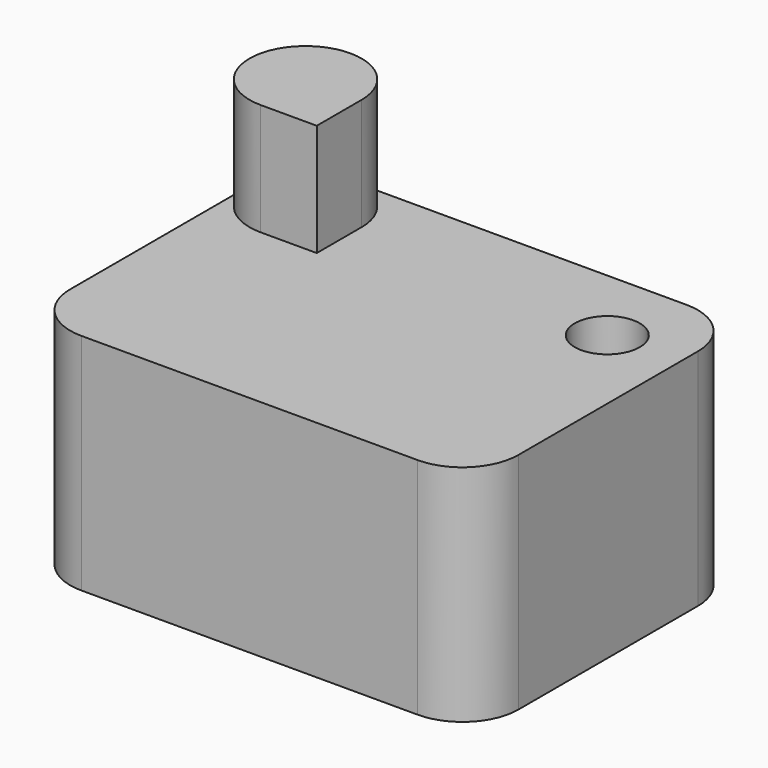
from build123d import *
from build123d import SkipClean  # not in build123d's __all__

# Parameters (mm, degrees)
F0_W      = 101.6
F0_H      = 76.2
F1_DEPTH  = 50.8
F2_R      = 12.7
F4_DEPTH  = 25.4
F9_R      = 7.3504137181
F10_DEPTH = 25.4


# Not quite as in the source:
# - after a boolean that leaves OpenCascade's solid faulty, fix() repairs it
# - the program builds the solid bodies; features that only make, move or delete a surface that nothing else refers to are left out


with BuildPart() as f1:
    # F0 (on Top) → F1 (new body)
    with BuildSketch(Plane.XY):
        with Locations((50.8, 38.1)):
            Rectangle(F0_W, F0_H)
    extrude(amount=F1_DEPTH)

    # F2
    f2_edges = [f1.edges().sort_by_distance(p)[0] for p in [
        (0, 0, 25.4),
        (101.6, 0, 25.4),
        (101.6, 76.2, 25.4),
        (0, 76.2, 25.4),
    ]]
    fillet(f2_edges, radius=F2_R)

    # F3 (on face) → F4 (join)
    with BuildSketch(Plane.XY.offset(50.8)):
        with BuildLine():
            ThreePointArc((0, 63.5), (3.7197438789, 54.5197438789), (12.7, 50.8))
            Line((12.7, 50.8), (25.4, 50.8))
            Line((25.4, 50.8), (25.4, 63.5))
            ThreePointArc((25.4, 63.5), (21.6802561211, 72.4802561211), (12.7, 76.2))
            ThreePointArc((12.7, 76.2), (3.7197438789, 72.4802561211), (0, 63.5))
        make_face()
    with SkipClean():  # cleaning this boolean's faces spoils the solid; the shape is the same uncleaned
        extrude(amount=F4_DEPTH)

    # F9 (on face) → F10 (cut)
    with BuildSketch(Plane.XY.offset(50.8)):
        with Locations((85.2179154754, 58.332465589)):
            Circle(F9_R)
    extrude(amount=-F10_DEPTH, mode=Mode.SUBTRACT)

    add(f1.part.fix(), mode=Mode.REPLACE)


solid = f1.part
